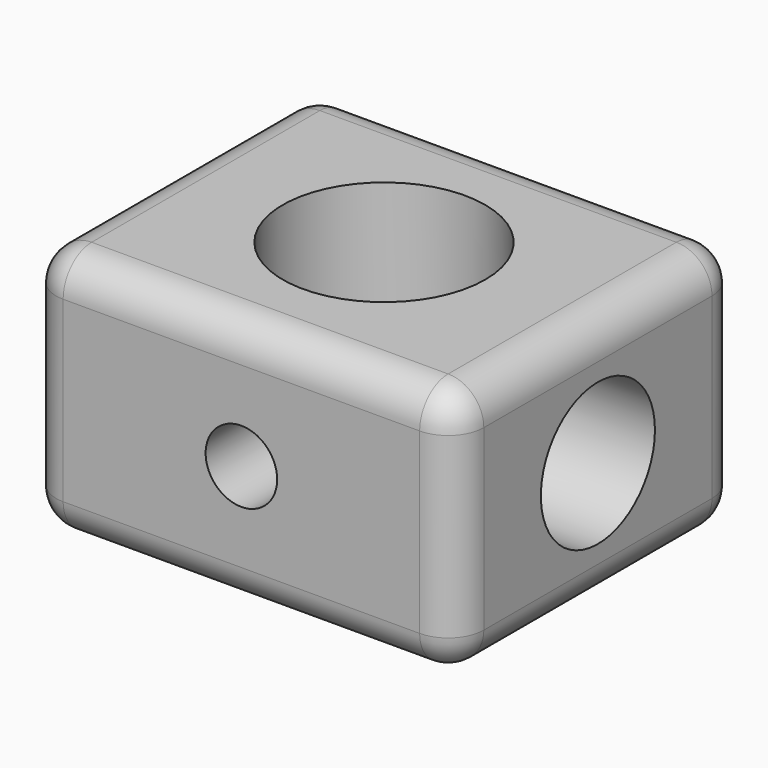
from build123d import *

# Parameters (mm, degrees)
F0_W     = 60
F0_H     = 50
F1_DEPTH = 35
F2_R     = 5
F3_R     = 10
F4_DEPTH = 30
F5_R     = 14.2018831862
F6_DEPTH = 30
F7_R     = 5.0166024016
F8_DEPTH = 13.3


# Not quite as in the source:
# - the program builds the solid bodies; features that only make, move or delete a surface that nothing else refers to are left out


with BuildPart() as f1:
    # F0 (on Top) → F1 (new body)
    with BuildSketch(Plane.XY):
        with Locations((-30, 25)):
            Rectangle(F0_W, F0_H)
    extrude(amount=F1_DEPTH)

    # F2
    f2_edges = [f1.edges().sort_by_distance(p)[0] for p in [
        (-60, 25, 35),
        (-30, 50, 35),
        (-30, 50, 0),
        (-60, 25, 0),
        (-60, 0, 17.5),
        (0, 50, 17.5),
        (-60, 50, 17.5),
        (0, 0, 17.5),
        (0, 25, 0),
        (0, 25, 35),
        (-30, 0, 35),
        (-30, 0, 0),
    ]]
    fillet(f2_edges, radius=F2_R)

    # F3 (on face) → F4 (cut)
    with BuildSketch(Plane.YZ):
        with Locations((25, 17.5)):
            Circle(F3_R)
    extrude(amount=-F4_DEPTH, mode=Mode.SUBTRACT)

    # F5 (on face) → F6 (cut)
    with BuildSketch(Plane.XY.offset(35)):
        with Locations((-30, 25)):
            Circle(F5_R)
    extrude(amount=-F6_DEPTH, mode=Mode.SUBTRACT)

    # F7 (on face) → F8 (cut)
    with BuildSketch(Plane.XZ):
        with Locations((-30, 17.5)):
            Circle(F7_R)
    extrude(amount=-F8_DEPTH, mode=Mode.SUBTRACT)


solid = f1.part
